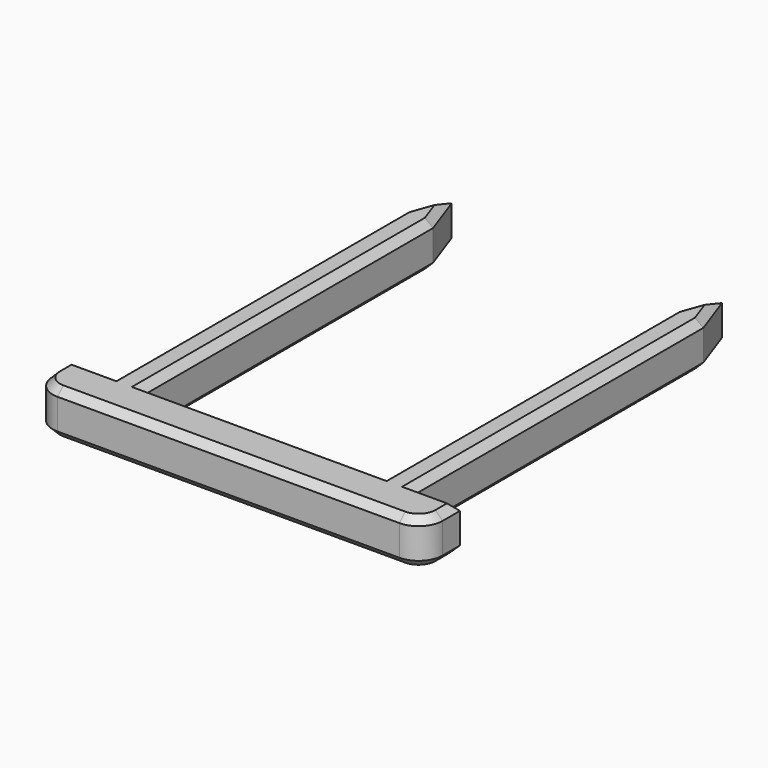
from build123d import *

# Parameters (mm, degrees)
F0_W     = 1.5748
F0_H     = 38.1
F1_DEPTH = 4.7498
F2_SIZE  = 0.762


# Not quite as in the source:
# - a feature names something its author has since deleted; it is built from what else it names


with BuildPart() as f1:
    # F0 (on Top) → F1 (new body)
    with BuildSketch(Plane.XY):
        with Locations((-11.2433909576, -6.3634803519)):
            Rectangle(F0_W, F0_H)
        with BuildLine():
            Line((-10.4559909576, -25.4134803519), (-12.0307909576, -25.4134803519))
            Line((-12.0307909576, -25.4134803519), (-12.0307909576, 12.6865196481))
            Line((-12.0307909576, 12.6865196481), (-12.0307909576, 17.1203389764))
            Line((-12.0307909576, 17.1203389764), (-13.6055909576, 12.6865196481))
            Line((-13.6055909576, 12.6865196481), (-13.6055909576, -25.4134803519))
            Line((-13.6055909576, -25.4134803519), (-18.3553909576, -25.4134803519))
            Line((-18.3553909576, -25.4134803519), (-18.3553909576, -27.7027830635))
            ThreePointArc((-18.3553909576, -27.7027830635), (-17.6114421818, -29.4988342878), (-15.8153909576, -30.2427830635))
            Line((-15.8153909576, -30.2427830635), (20.3288090424, -30.2427830635))
            ThreePointArc((20.3288090424, -30.2427830635), (22.1248602666, -29.4988342878), (22.8688090424, -27.7027830635))
            Line((22.8688090424, -27.7027830635), (22.8688090424, -25.4134803519))
            Line((22.8688090424, -25.4134803519), (18.1190090424, -25.4134803519))
            Line((18.1190090424, -25.4134803519), (18.1190090424, 12.6865196481))
            Line((18.1190090424, 12.6865196481), (16.5442090424, 17.1203389764))
            Line((16.5442090424, 17.1203389764), (16.5442090424, 12.6865196481))
            Line((16.5442090424, 12.6865196481), (16.5442090424, -25.4134803519))
            Line((16.5442090424, -25.4134803519), (14.9694090424, -25.4134803519))
            Line((14.9694090424, -25.4134803519), (-10.4559909576, -25.4134803519))
        make_face()
        with Locations((15.7568090424, -6.3634803519)):
            Rectangle(F0_W, F0_H)
        Polygon((-12.0307909576, 17.1203389764), (-12.0307909576, 12.6865196481), (-10.4559909576, 12.6865196481), align=None)
        Polygon((16.5442090424, 17.1203389764), (14.9694090424, 12.6865196481), (16.5442090424, 12.6865196481), align=None)
    extrude(amount=F1_DEPTH)

    # F2
    f2_edges = [f1.edges().sort_by_distance(p)[0] for p in [
        (-13.605591, -6.36348, 4.7498),
        (-10.455991, -6.36348, 4.7498),
        (-11.243391, 14.903429, 4.7498),
        (-12.818191, 14.903429, 4.7498),
        (-15.980491, -25.41348, 4.7498),
        (-18.355391, -26.558132, 4.7498),
        (-17.611442, -29.498834, 4.7498),
        (2.256709, -30.242783, 4.7498),
        (22.12486, -29.498834, 4.7498),
        (22.868809, -26.558132, 4.7498),
        (20.493909, -25.41348, 4.7498),
        (18.119009, -6.36348, 4.7498),
        (17.331609, 14.903429, 4.7498),
        (15.756809, 14.903429, 4.7498),
        (14.969409, -6.36348, 4.7498),
        (2.256709, -25.41348, 4.7498),
        (-10.455991, -6.36348, 0),
        (-11.243391, 14.903429, 0),
        (-12.818191, 14.903429, 0),
        (-13.605591, -6.36348, 0),
        (-15.980491, -25.41348, 0),
        (-18.355391, -26.558132, 0),
        (-17.611442, -29.498834, 0),
        (2.256709, -30.242783, 0),
        (22.12486, -29.498834, 0),
        (22.868809, -26.558132, 0),
        (20.493909, -25.41348, 0),
        (18.119009, -6.36348, 0),
        (17.331609, 14.903429, 0),
        (15.756809, 14.903429, 0),
        (14.969409, -6.36348, 0),
        (2.256709, -25.41348, 0),
    ]]
    chamfer(f2_edges, length=F2_SIZE)


solid = f1.part
